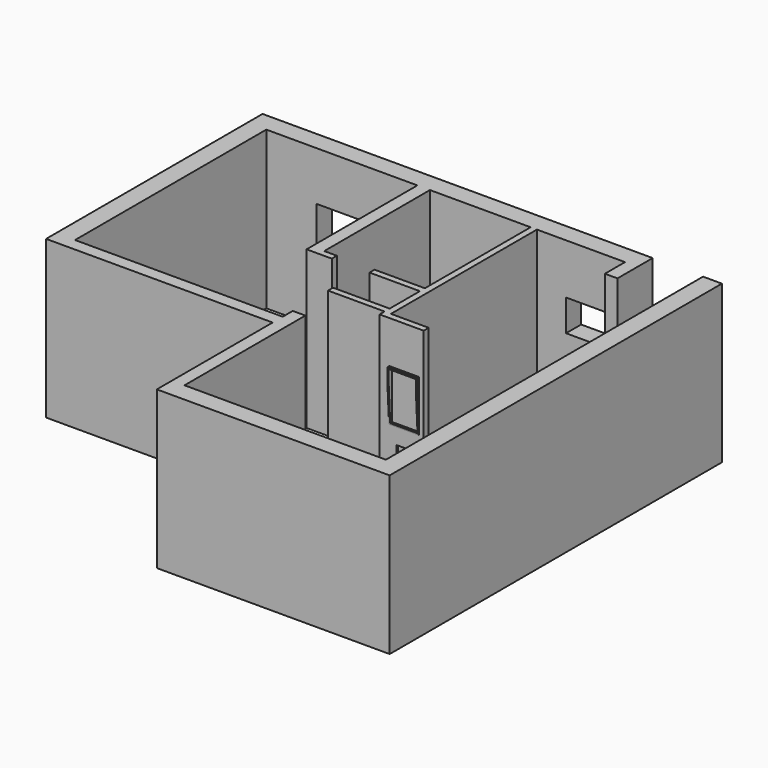
from build123d import *

# Parameters (mm, degrees)
F0_W      = 3300
F0_H      = 200
F0_W_2    = 300
F0_H_2    = 5600
F0_H_3    = 700
F0_W_3    = 900
F0_H_4    = 100
F0_W_4    = 800
F0_W_5    = 200
F0_H_5    = 2100
F1_DEPTH  = 2500
F2_W      = 1000
F2_H      = 600
F2_W_2    = 800
F2_H_2    = 500
F2_W_3    = 398.3602523804
F2_H_3    = 494.5161342621
F3_DEPTH  = 990
F4_W      = 240
F4_H      = 420
F4_W_2    = 474
F4_H_2    = 808
F5_DEPTH  = 30
F6_W      = 474
F6_H      = 20
F7_DEPTH  = 40
F8_W      = 474
F8_H      = 20
F9_DEPTH  = 70
F11_DEPTH = 20
F12_START = 454
F12_DEPTH = 20


with BuildPart() as f1:
    # F0 (on Top) → F1 (new body)
    with BuildSketch(Plane.XY):
        Polygon((-7000, 400), (-6700, 400), (-4300, 400), (-4100, 400), (-2500, 400), (-2400, 400), (-1000, 400), (-1000, 700), (-7000, 700), align=None)
        Polygon((-7000, -3600), (-6700, -3600), (-6700, -3400), (-6700, 400), (-7000, 400), align=None)
        with Locations((-5050, -3500)):
            Rectangle(F0_W, F0_H)
        Polygon((-3200, -5900), (-3200, -5600), (-3200, -3200), (-3400, -3200), (-3400, -3400), (-3400, -3600), (-3400, -5900), align=None)
        Polygon((300, -5600), (0, -5600), (-3200, -5600), (-3200, -5900), (300, -5900), align=None)
        with Locations((150, -2800)):
            Rectangle(F0_W_2, F0_H_2)
        with Locations((150, 350)):
            Rectangle(F0_W_2, F0_H_3)
        Polygon((-800, 700), (-1000, 700), (-1000, 400), (-1000, 0), (-800, 0), align=None)
        Polygon((-1800, -2500), (-2400, -2500), (-2500, -2500), (-2500, -2600), (-1800, -2600), align=None)
        Polygon((-2400, 400), (-2500, 400), (-2500, -1700), (-2500, -1800), (-2500, -2400), (-2500, -2500), (-2400, -2500), align=None)
        with Locations((-2950, -2450)):
            Rectangle(F0_W_3, F0_H_4)
        with Locations((-2900, -1750)):
            Rectangle(F0_W_4, F0_H_4)
        with Locations((-4000, -1750)):
            Rectangle(F0_W_5, F0_H_4)
        with Locations((-4200, -1750)):
            Rectangle(F0_W_5, F0_H_4)
        with Locations((-4200, -650)):
            Rectangle(F0_W_5, F0_H_5)
    extrude(amount=F1_DEPTH)

    # F2 (on face) → F3 (cut)
    with BuildSketch(Plane(origin=(0, 700, 0), x_dir=(-1, 0, 0), z_dir=(0, 1, 0))):
        with Locations((5400, 1420.9607362747)):
            Rectangle(F2_W, F2_H)
        with Locations((1537.3227357864, 1450)):
            Rectangle(F2_W_2, F2_H_2)
        with Locations((2930.5288791656, 1524.4877338409)):
            Rectangle(F2_W_3, F2_H_3)
    extrude(amount=-F3_DEPTH, mode=Mode.SUBTRACT)

    # F4 (on face) → F5 (cut)
    with BuildSketch(Plane.XZ.offset(2600)):
        with Locations((-2110, 550)):
            Rectangle(F4_W, F4_H)
        with Locations((-2107, 1424)):
            Rectangle(F4_W_2, F4_H_2)
    extrude(amount=-F5_DEPTH, mode=Mode.SUBTRACT)


with BuildPart() as f7:
    # F6 (on face) → F7 (new body)
    with BuildSketch(Plane.XZ.offset(2570)):
        with Locations((-2107, 1030)):
            Rectangle(F6_W, F6_H)
    extrude(amount=F7_DEPTH)

    # F10 (on face) → F11 (join)
    with BuildSketch(Plane.YZ.offset(-2344)):
        Polygon((-2640.0933265686, 1608), (-2609.5175743103, 1040), (-2570, 1040), (-2570, 1808), (-2640.0933265686, 1808), align=None)
    extrude(amount=F11_DEPTH)

    # F10 (on face) → F12 (join)
    with BuildSketch(Plane.YZ.offset(-2344).offset(F12_START)):
        Polygon((-2640.0933265686, 1608), (-2609.5175743103, 1040), (-2570, 1040), (-2570, 1808), (-2640.0933265686, 1808), align=None)
    extrude(amount=F12_DEPTH)


with BuildPart() as f9:
    # F8 (on face) → F9 (new body)
    with BuildSketch(Plane.XZ.offset(2570)):
        with Locations((-2107, 1818)):
            Rectangle(F8_W, F8_H)
    extrude(amount=F9_DEPTH)


solid = Compound([f1.part, f7.part, f9.part])
